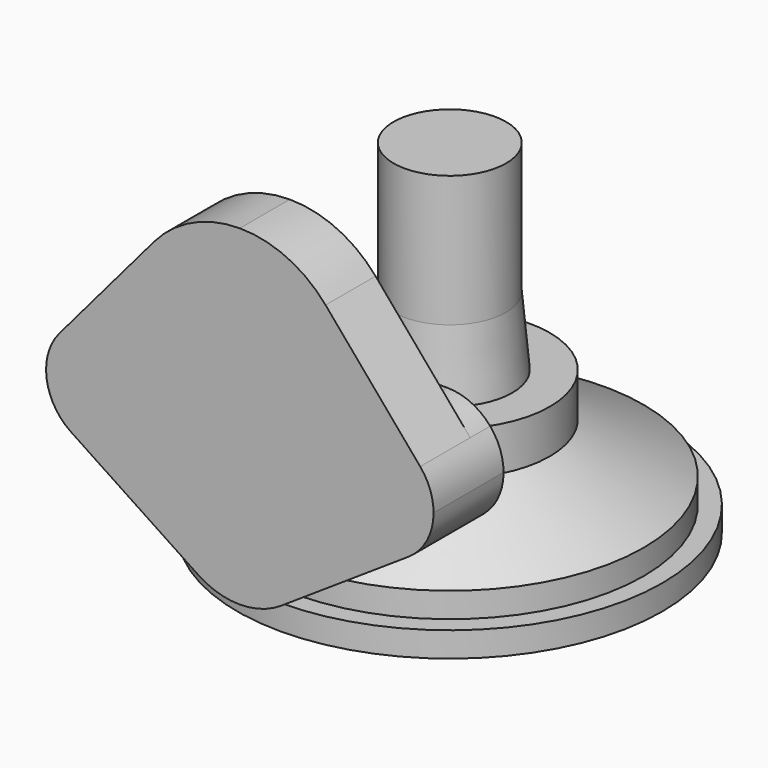
from build123d import *

# Parameters (mm, degrees)
F4_DEPTH = 14
F6_DEPTH = 4


with BuildPart() as f1:
    # F0 (on Front) → F1 (revolve)
    with BuildSketch(Plane.XZ):
        Polygon((0, 0), (34, 0), (34, 4), (31, 4), (31, 8), (16, 16), (16, 23), (10, 23), (9, 34), (9, 55), (0, 55), align=None)
    revolve(axis=Axis((0, 0, 27.5), (0, 0, -1)))


with BuildPart() as f4:
    # F3 (on offset) → F4 (new body)
    with BuildSketch(Plane.XZ.offset(42)):
        with BuildLine():
            ThreePointArc((26.9766909288, 22.501163597), (29.93064368, 25.7450157673), (31, 30))
            ThreePointArc((31, 30), (30.4480034885, 33.1034234416), (28.8597250983, 35.8261626802))
            Line((28.8597250983, 35.8261626802), (13.7194501966, 53.6523253604))
            ThreePointArc((13.7194501966, 53.6523253604), (7.5583775876, 58.3361846293), (0, 60))
            ThreePointArc((0, 60), (-7.5583775876, 58.3361846293), (-13.7194501966, 53.6523253604))
            Line((-13.7194501966, 53.6523253604), (-28.8597250983, 35.8261626802))
            ThreePointArc((-28.8597250983, 35.8261626802), (-30.4480034885, 33.1034234416), (-31, 30))
            ThreePointArc((-31, 30), (-29.93064368, 25.7450157673), (-26.9766909288, 22.501163597))
            Line((-26.9766909288, 22.501163597), (-6.635587905, 9.0015514626))
            ThreePointArc((-6.635587905, 9.0015514626), (-3.4654449607, 7.5112798265), (0, 7))
            ThreePointArc((0, 7), (3.4654449607, 7.5112798265), (6.635587905, 9.0015514626))
            Line((6.635587905, 9.0015514626), (26.9766909288, 22.501163597))
        make_face()
    extrude(amount=-F4_DEPTH)

    # F5 (on face) → F6 (cut)
    with BuildSketch(Plane(origin=(0, -28, 0), x_dir=(-1, 0, 0), z_dir=(0, 1, 0))):
        with BuildLine():
            ThreePointArc((-22, 21), (-24.5990837205, 21.3834598699), (-26.9766909288, 22.501163597))
            Line((-26.9766909288, 22.501163597), (-6.635587905, 9.0015514626))
            ThreePointArc((-6.635587905, 9.0015514626), (0, 7), (6.635587905, 9.0015514626))
            Line((6.635587905, 9.0015514626), (26.9766909288, 22.501163597))
            ThreePointArc((26.9766909288, 22.501163597), (24.5990837205, 21.3834598699), (22, 21))
            Line((22, 21), (-22, 21))
        make_face()
        with BuildLine():
            ThreePointArc((-28.8597250983, 35.8261626802), (-25.7791887938, 38.1680923147), (-22, 39))
            Line((-22, 39), (22, 39))
            ThreePointArc((22, 39), (25.7791887938, 38.1680923147), (28.8597250983, 35.8261626802))
            Line((28.8597250983, 35.8261626802), (13.7194501966, 53.6523253604))
            ThreePointArc((13.7194501966, 53.6523253604), (0, 60), (-13.7194501966, 53.6523253604))
            Line((-13.7194501966, 53.6523253604), (-28.8597250983, 35.8261626802))
        make_face()
    extrude(amount=-F6_DEPTH, mode=Mode.SUBTRACT)


solid = Compound([f1.part, f4.part])
